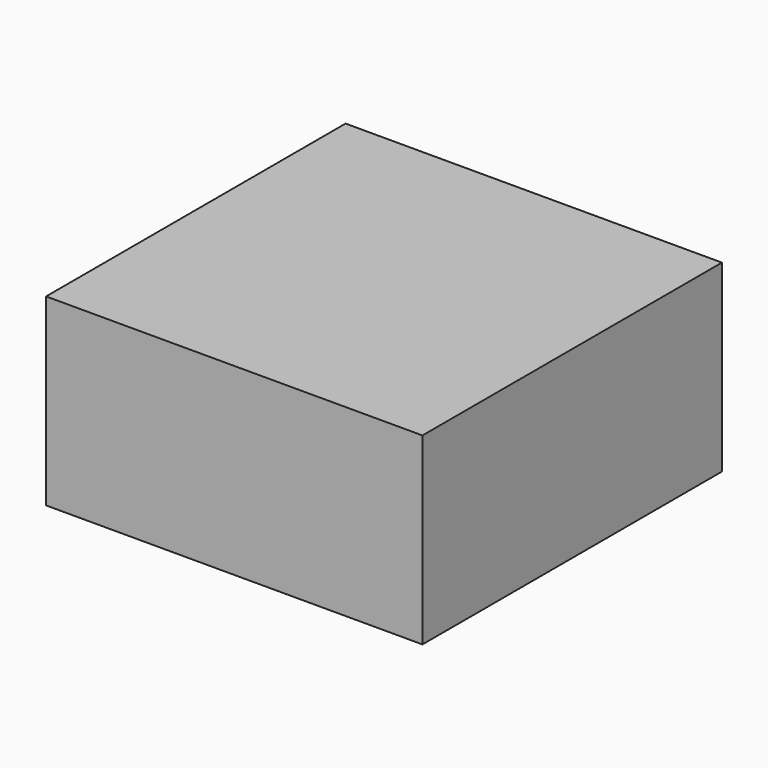
from build123d import *

# Parameters (mm, degrees)
F0_W     = 128.847271204
F0_H     = 128.1545460224
F4_DEPTH = 62.992


# Not quite as in the source:
# - the program builds the solid bodies; features that only make, move or delete a surface that nothing else refers to are left out


with BuildPart() as f4:
    # F0 (on Top) → F4 (new body)
    with BuildSketch(Plane.XY):
        Rectangle(F0_W, F0_H)
    extrude(amount=-F4_DEPTH)


solid = f4.part
